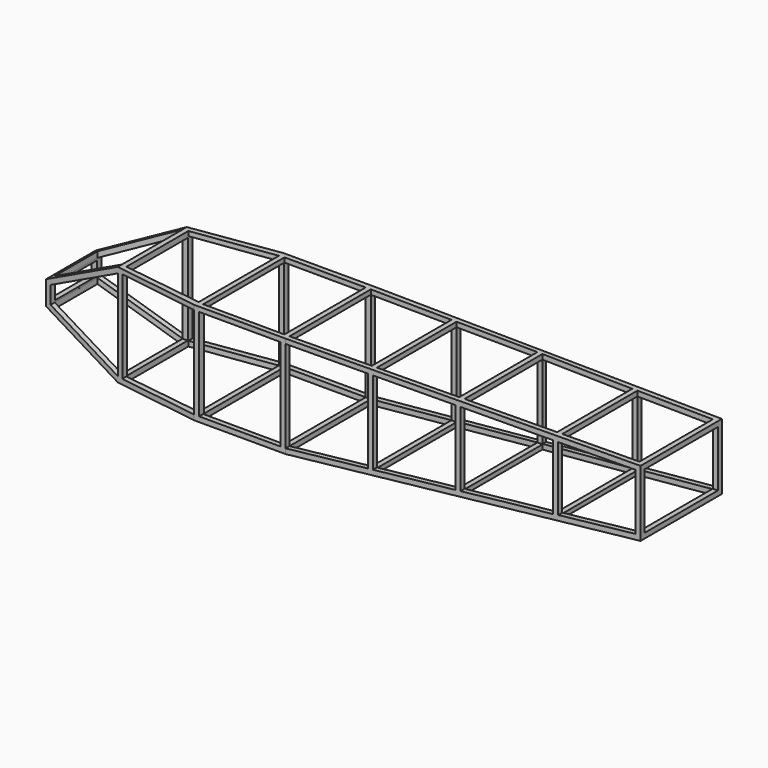
from build123d import *

# Parameters (mm, degrees)
F0_W      = 1524
F0_H      = 355.6
F2_DEPTH  = 127
F5_W      = 12.7
F5_H      = 295.684620738
F6_DEPTH  = 177.8
F8_DEPTH  = 190.5
F9_W      = 1716.6963219643
F9_H      = 471.6365635395
F10_DEPTH = 190.5
F12_DEPTH = 190.5
F13_W     = 1570.3657865524
F13_H     = 143.7467932701
F14_DEPTH = 190.5
F15_W     = 189.6323112059
F15_H     = 225.8323701404
F16_DEPTH = 25.4
F17_W     = 250.2110230158
F17_H     = 229.754279344
F18_DEPTH = 25.4
F19_W     = 254.0152243916
F19_H     = 229.5392287665
F20_DEPTH = 25.4
F21_W     = 248.717826187
F21_H     = 208.6506967284
F22_DEPTH = 25.4
F23_W     = 244.0285278141
F23_H     = 186.4718558426
F24_DEPTH = 15.24
F25_W     = 234.5546834328
F25_H     = 162.4008728846
F26_DEPTH = 13.97
F28_W     = 129.7433354616
F28_H     = 34.350046491
F29_DEPTH = 25.4
F30_W     = 228.6
F30_H     = 139.7
F31_DEPTH = 12.7


# Not quite as in the source:
# - a feature names something its author has since deleted; it is built from what else it names


with BuildPart() as f2:
    # F0 (on Top) → F2 (new body, symmetric)
    with BuildSketch(Plane.XY):
        Rectangle(F0_W, F0_H)
    extrude(amount=F2_DEPTH, both=True)

    # F5 (on Front) → F6 (join, symmetric)
    with BuildSketch(Plane.XZ):
        with Locations((-552.45, 4.7732368112)):
            Rectangle(F5_W, F5_H)
        with Locations((-336.55, 4.7732368112)):
            Rectangle(F5_W, F5_H)
        with Locations((-120.65, 4.7732368112)):
            Rectangle(F5_W, F5_H)
        with Locations((95.25, 4.7732368112)):
            Rectangle(F5_W, F5_H)
        with Locations((552.45, 4.7732368112)):
            Rectangle(F5_W, F5_H)
        with Locations((311.15, 4.7732368112)):
            Rectangle(F5_W, F5_H)
    extrude(amount=F6_DEPTH, both=True)

    # F7 (on Front) → F8 (cut, symmetric)
    with BuildSketch(Plane.XZ):
        Polygon((-1015.0121382617, 307.3465449898), (-843.425049348, -20.5651363992), (-558.8, 127), align=None)
        Polygon((-558.8, -127), (-762, -38.1), (-810.4430437088, -38.1), (-810.4430437088, -218.054279685), (819.7100162506, -218.054279685), (819.7100162506, -38.1), (762, -38.1), (-114.3, -127), align=None)
    extrude(amount=F8_DEPTH, both=True, mode=Mode.SUBTRACT)

    # F9 (on Top) → F10 (cut, symmetric)
    with BuildSketch(Plane.XY):
        with Locations((-0.0626146793, 9.3713402748)):
            Rectangle(F9_W, F9_H)
        Polygon((762, 127), (762, 0), (762, -127), (-114.3, -139.7), (-342.9, -139.7), (-762, -77.5716677308), (-762, 0), (-762, 77.5716677308), (-342.9, 139.7), (-114.3, 139.7), align=None, mode=Mode.SUBTRACT)
    extrude(amount=F10_DEPTH, both=True, mode=Mode.SUBTRACT)

    # F11 (on Top) → F12 (cut, symmetric)
    with BuildSketch(Plane.XY):
        Polygon((-749.2891273529, 66.8201254906), (-749.2891273529, -66.6171684709), (-558.8, -94.8557077165), (-558.8, 94.7766034894), align=None)
        Polygon((749.3002457909, -114.4827207254), (749.3002457909, 114.4827207254), (558.8, 117.2435938528), (558.8, -117.2435938528), align=None)
        Polygon((-127, -127.6207012333), (-127, 126.3945231583), (-330.2, 126.8815944692), (-330.2, -126.8815944692), align=None)
        Polygon((-546.1, -96.6881841261), (-342.9, -125.1055115079), (-342.9, 125.1055115079), (-546.1, 96.6881841261), align=None)
        Polygon((88.9, -124.4917157261), (88.9, 124.226110461), (-114.3, 126.3945231583), (-114.3, -127.4366432623), align=None)
        Polygon((101.6, 124.0527423648), (101.6, -124.3076577551), (304.8, -121.3627302188), (304.8, 122.6657975952), align=None)
        Polygon((317.5, 122.4924294991), (317.5, -120.8313876883), (546.1, -117.4366649156), (546.1, 117.1180185172), align=None)
    extrude(amount=F12_DEPTH, both=True, mode=Mode.SUBTRACT)

    # F13 (on Front) → F14 (cut, symmetric)
    with BuildSketch(Plane.XZ):
        Polygon((-558.8, 112.6946179402), (-749.3, 13.9290365255), (-749.3, -29.7940022002), (-558.8, -113.1377522002), align=None)
        Polygon((-546.1, -114.3), (-342.9, -114.3), (-342.9, 115.454279344), (-546.1, 115.7130942238), align=None)
        Polygon((558.8, -45.9493061315), (749.3, -26.623219175), (749.3, 114.3), (558.8, 114.3), align=None)
        Polygon((-330.2, -114.303525896), (-127, -114.3599402323), (-127, 115.1792885342), (-330.2, 115.438103414), align=None)
        Polygon((304.8, 114.6293069146), (101.6, 114.8881217944), (101.6, -92.4570416816), (304.8, -71.842548928), align=None)
        Polygon((456.2991908124, -56.4730658021), (546.1, -48.1008728846), (546.1, 114.3), (317.5, 114.6119749718), (317.5, -70.5541431309), align=None)
        with Locations((66.4489865303, 198.8733966351)):
            Rectangle(F13_W, F13_H)
        Polygon((-114.3, 115.1792885342), (-114.3, -114.3599402323), (88.9, -93.7454474787), (88.9, 114.9052492497), align=None)
    extrude(amount=F14_DEPTH, both=True, mode=Mode.SUBTRACT)

    # F15 (on face) → F16 (cut)
    with BuildSketch(Plane(origin=(-558.8, 0, 0), x_dir=(0, -1, 0), z_dir=(-1, 0, 0))):
        with Locations((0.0395521135, -0.22156713)):
            Rectangle(F15_W, F15_H)
    extrude(amount=-F16_DEPTH, mode=Mode.SUBTRACT)

    # F17 (on face) → F18 (cut)
    with BuildSketch(Plane(origin=(-342.9, 0, 0), x_dir=(0, -1, 0), z_dir=(-1, 0, 0))):
        with Locations((0, 0.577139672)):
            Rectangle(F17_W, F17_H)
    extrude(amount=-F18_DEPTH, mode=Mode.SUBTRACT)

    # F19 (on face) → F20 (cut)
    with BuildSketch(Plane(origin=(-127, 0, 0), x_dir=(0, -1, 0), z_dir=(-1, 0, 0))):
        with Locations((0.6130890375, 0.4096741509)):
            Rectangle(F19_W, F19_H)
    extrude(amount=-F20_DEPTH, mode=Mode.SUBTRACT)

    # F21 (on face) → F22 (cut)
    with BuildSketch(Plane(origin=(88.9, 0, 0), x_dir=(0, -1, 0), z_dir=(-1, 0, 0))):
        with Locations((0.1328026326, 10.5799008855)):
            Rectangle(F21_W, F21_H)
    extrude(amount=-F22_DEPTH, mode=Mode.SUBTRACT)

    # F23 (on face) → F24 (cut)
    with BuildSketch(Plane(origin=(304.8, 0, 0), x_dir=(0, -1, 0), z_dir=(-1, 0, 0))):
        with Locations((-0.6515336882, 21.3933789933)):
            Rectangle(F23_W, F23_H)
    extrude(amount=-F24_DEPTH, mode=Mode.SUBTRACT)

    # F25 (on face) → F26 (cut)
    with BuildSketch(Plane(origin=(546.1, 0, 0), x_dir=(0, -1, 0), z_dir=(-1, 0, 0))):
        with Locations((0.1593231992, 33.0995635577)):
            Rectangle(F25_W, F25_H)
    extrude(amount=-F26_DEPTH, mode=Mode.SUBTRACT)

    # F28 (on face) → F29 (cut)
    with BuildSketch(Plane(origin=(-762, 0, 0), x_dir=(0, -1, 0), z_dir=(-1, 0, 0))):
        with Locations((0, -8.2249767545)):
            Rectangle(F28_W, F28_H)
    extrude(amount=-F29_DEPTH, mode=Mode.SUBTRACT)

    # F30 (on face) → F31 (cut)
    with BuildSketch(Plane.YZ.offset(762)):
        with Locations((0, 44.45)):
            Rectangle(F30_W, F30_H)
    extrude(amount=-F31_DEPTH, mode=Mode.SUBTRACT)


solid = f2.part
